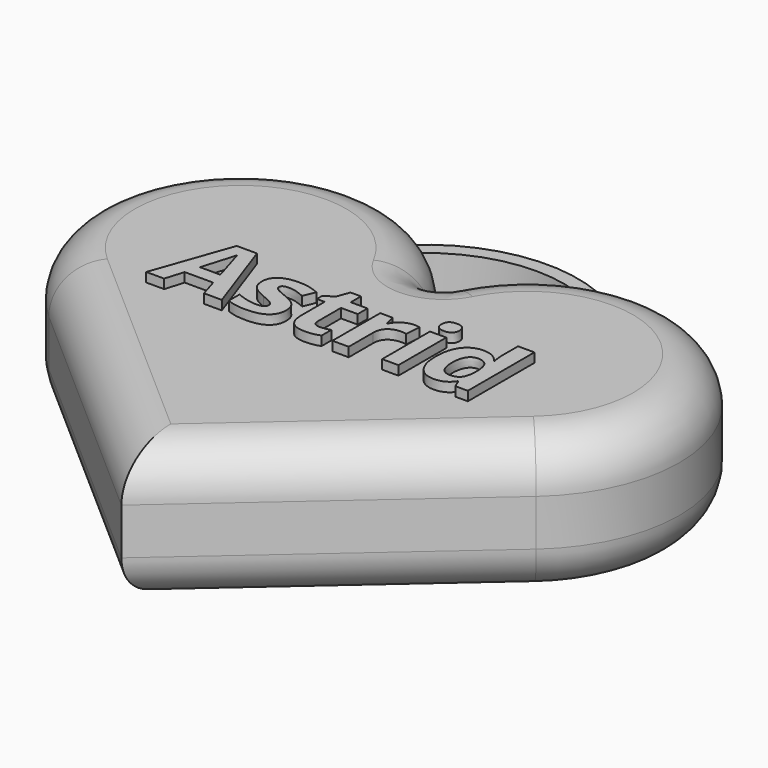
from build123d import *

# Parameters (mm, degrees)
F1_DEPTH      = 30
F4_DEPTH      = 4
F4_DEPTH_BACK = 4
F5_R          = 2
F6_R          = 10
F7_TEXT_SIZE  = 23.6061142964
F8_DEPTH      = 2


# Not quite as in the source:
# - Text() gives the source's letters only with a copy of the font that has no kerning and outlines rounded to 1/6400 em; it was checked with that copy


with BuildPart() as f1:
    # F0 (on Top) → F1 (new body)
    with BuildSketch(Plane.XY):
        with BuildLine():
            Line((0, -46.0824511092), (52.5109021469, 0))
            ThreePointArc((52.5109021469, 0), (49.304363297, 51.7701212776), (0, 35.6608969519))
            ThreePointArc((0, 35.6608969519), (-49.304363297, 51.7701212776), (-52.5109021469, 0))
            Line((-52.5109021469, 0), (0, -46.0824511092))
        make_face()
    extrude(amount=F1_DEPTH)

    # F3 (on mid) → F4 (join, two sides)
    with BuildSketch(Plane.XY.offset(15)) as f4_sk:
        with BuildLine():
            ThreePointArc((-21.8888995597, 56.1761614168), (0, 65.6608969519), (21.8888995597, 56.1761614168))
            ThreePointArc((21.8888995597, 56.1761614168), (23.5453632224, 56.6022750201), (25.2217932497, 56.9414313735))
            ThreePointArc((25.2217932497, 56.9414313735), (0, 68.6608969519), (-25.2217932497, 56.9414313735))
            ThreePointArc((-25.2217932497, 56.9414313735), (-23.5453632224, 56.6022750201), (-21.8888995597, 56.1761614168))
        make_face()
    extrude(amount=F4_DEPTH)
    extrude(f4_sk.sketch, amount=-F4_DEPTH_BACK)

    # F5
    f5_edges = [f1.edges().sort_by_distance(p)[0] for p in [
        (0, 35.660897, 15),
    ]]
    fillet(f5_edges, radius=F5_R)

    # F6
    f6_edges = [f1.edges().sort_by_distance(p)[0] for p in [
        (-51.102076, 50.457961, 30),
        (-51.102076, 50.457961, 0),
    ]]
    fillet(f6_edges, radius=F6_R)

    # F7 (on face) → F8 (join)
    with BuildSketch(Plane.XY.offset(30)):
        with Locations((-35.4128599, 4.8774201423)):
            Text('Astrid', F7_TEXT_SIZE, font='Open Sans', font_style=FontStyle.BOLD, text_align=(TextAlign.LEFT, TextAlign.BOTTOM))
    extrude(amount=F8_DEPTH)


solid = f1.part
